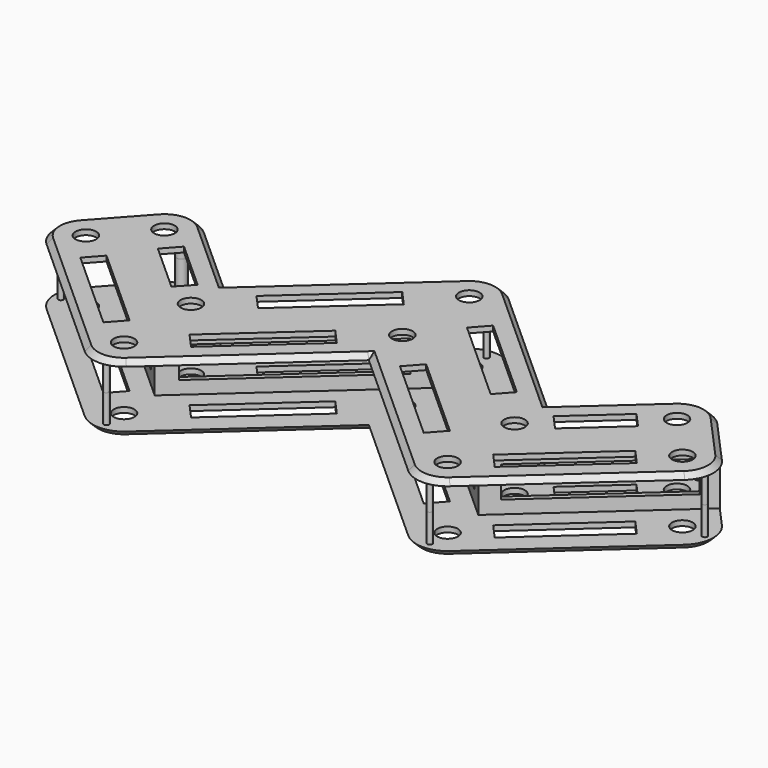
from build123d import *

# Parameters (mm, degrees)
F0_R           = 2
F0_R_2         = 1
F0_R_3         = 0.5
F1_DEPTH       = 6.5
F2_DEPTH       = 5.5
F3_W           = 30
F3_H           = 6
F4_DEPTH       = 1
F5_W           = 35
F5_H           = 6
F6_DEPTH       = 1.5
F7_W           = 35
F7_H           = 6
F8_DEPTH       = 1.5
F9_W           = 30
F9_H           = 6
F10_DEPTH      = 1.5
F11_R          = 6
F12_DEPTH      = 6.5
F13_T1_DEPTH   = 35.4024242658
F13_T3_DEPTH   = 35.4024242658
F13_T5_DEPTH   = 12
F13_T7_DEPTH   = 12
F13_T10_ANGLE  = 84
F13_T14_DEPTH  = 39.1692587222
F13_T19_DEPTH  = 39.1692587222
F13_T22_ANGLE  = 84
F13_T24_ANGLE  = 90
F13_T26_ANGLE  = 90
F13_T30_DEPTH  = 21.7668344564
F13_T35_DEPTH  = 39.1692587222
F13_T38_ANGLE  = 84
F13_T42_DEPTH  = 39.1692587222
F13_T47_DEPTH  = 21.7668344564
F13_T50_ANGLE  = 90
F13_T52_ANGLE  = 90
F13_T54_ANGLE  = 90
F13_T56_ANGLE  = 90
F13_T60_DEPTH  = 21.7668344564
F13_T65_DEPTH  = 39.1692587222
F13_T68_ANGLE  = 84
F13_T72_DEPTH  = 39.1692587222
F13_T77_DEPTH  = 21.7668344564
F13_T80_ANGLE  = 90
F13_T82_ANGLE  = 90
F13_T84_ANGLE  = 84
F13_T88_DEPTH  = 39.1692587222
F13_T93_DEPTH  = 39.1692587222
F13_T96_ANGLE  = 84
F13_T101_DEPTH = 39.1692587222
F13_T105_DEPTH = 39.1692587222
F13_T112_DEPTH = 21.7668344564
F13_T116_DEPTH = 39.1692587222
F13_T123_DEPTH = 39.1692587222
F13_T127_DEPTH = 21.7668344564
F13_T134_DEPTH = 21.7668344564
F13_T138_DEPTH = 39.1692587222
F13_T145_DEPTH = 39.1692587222
F13_T149_DEPTH = 21.7668344564
F13_T156_DEPTH = 39.1692587222
F13_T160_DEPTH = 39.1692587222


# Not quite as in the source:
# - a fillet or chamfer that OpenCascade refuses, or shapes differently, is made with other operations: its cross-section is extruded or revolved along the edge and cut away or added


with BuildPart() as f1:
    # F0 (on Top) → F1 (new body, symmetric)
    with BuildSketch(Plane.XY):
        Polygon((-49.9357291109, 33.0064397346), (-57.6307310841, 24.4602742417), (-31.2120826701, 0.6728163648), (0, 28.7763018319), (31.2120826701, 0.6728163648), (57.6307310841, 24.4602742417), (49.9357291109, 33.0064397346), (31.2120826701, 16.1475927553), (0, 44.2510782223), (-31.2120826701, 16.1475927553), align=None)
        with Locations((-31.2120826701, 8.0737963776)):
            Circle(F0_R, mode=Mode.SUBTRACT)
        with Locations((31.2120826701, 8.0737963776)):
            Circle(F0_R, mode=Mode.SUBTRACT)
        Polygon((-46.3710360561, 19.0317138545), (-43.6945136306, 22.0042931564), (-34.3115040691, 13.5557933995), (-37.0313460748, 10.6222192229), align=None, mode=Mode.SUBTRACT)
        with Locations((-49.8654209077, 29.0960744023)):
            Circle(F0_R_2, mode=Mode.SUBTRACT)
        with Locations((-49.4916437962, 24.5327871436)):
            Circle(F0_R, mode=Mode.SUBTRACT)
        Polygon((-22.4423732026, 13.2788127903), (-25.118895628, 16.2513920922), (-8.7697094675, 30.9722654321), (-6.0931870421, 27.9996861302), align=None, mode=Mode.SUBTRACT)
        Polygon((6.0931870421, 27.9996861302), (8.7697094675, 30.9722654321), (25.118895628, 16.2513920922), (22.4423732026, 13.2788127903), align=None, mode=Mode.SUBTRACT)
        Polygon((37.0092128356, 10.6022903648), (34.3326904102, 13.5748696667), (43.6361429708, 21.9517359782), (46.3126653962, 18.9791566763), align=None, mode=Mode.SUBTRACT)
        with Locations((49.4332731364, 24.4802299654)):
            Circle(F0_R, mode=Mode.SUBTRACT)
        with Locations((0, 36.1772818447)):
            Circle(F0_R, mode=Mode.SUBTRACT)
        with Locations((0, 40.3471924365)):
            Circle(F0_R_3, mode=Mode.SUBTRACT)
        with Locations((49.6616996825, 29.187746346)):
            Circle(F0_R_3, mode=Mode.SUBTRACT)
        Polygon((-31.2120826701, -0.6728163648), (-58.2998616904, 23.7171294162), (-65.9948636635, 15.1709639232), (-31.2120826701, -16.1475927553), (0, 11.9558927118), (31.2120826701, -16.1475927553), (65.9948636635, 15.1709639232), (58.2998616904, 23.7171294162), (31.2120826701, -0.6728163648), (0, 27.4306691023), align=None)
        with Locations((-31.124683097, -12.420842424)):
            Circle(F0_R_3, mode=Mode.SUBTRACT)
        with Locations((-31.2120826701, -8.0737963776)):
            Circle(F0_R, mode=Mode.SUBTRACT)
        Polygon((-53.6574585069, 9.4448453424), (-50.9809360815, 12.4174246443), (-35.0758352357, -1.9035924822), (-37.7523576611, -4.8761717841), align=None, mode=Mode.SUBTRACT)
        Polygon((-6.0931870421, 11.8520933749), (-22.4423732026, -2.868779965), (-25.118895628, 0.1037993369), (-8.7697094675, 14.8246726768), align=None, mode=Mode.SUBTRACT)
        with Locations((31.263994053, -12.4030448496)):
            Circle(F0_R_3, mode=Mode.SUBTRACT)
        with Locations((31.2120826701, -8.0737963776)):
            Circle(F0_R, mode=Mode.SUBTRACT)
        Polygon((22.4423732026, -2.868779965), (6.0931870421, 11.8520933749), (8.7697094675, 14.8246726768), (25.118895628, 0.1037993369), align=None, mode=Mode.SUBTRACT)
        Polygon((37.7523576611, -4.8761717841), (35.0758352357, -1.9035924822), (51.0113683193, 12.4448259544), (53.6878907447, 9.4722466525), align=None, mode=Mode.SUBTRACT)
        with Locations((-61.948928982, 15.132994391)):
            Circle(F0_R_3, mode=Mode.SUBTRACT)
        with Locations((-57.5212110725, 15.6150492379)):
            Circle(F0_R, mode=Mode.SUBTRACT)
        with Locations((0, 20.0296890894)):
            Circle(F0_R, mode=Mode.SUBTRACT)
        with Locations((57.5516433104, 15.6424505479)):
            Circle(F0_R, mode=Mode.SUBTRACT)
        with Locations((62.0999746025, 15.3564941138)):
            Circle(F0_R_3, mode=Mode.SUBTRACT)
        Polygon((-57.6307310841, 24.4602742417), (-57.9652963872, 24.0887018289), (-31.2120826701, 0), (0, 28.1034854671), (31.2120826701, 0), (57.9652963872, 24.0887018289), (57.6307310841, 24.4602742417), (31.2120826701, 0.6728163648), (0, 28.7763018319), (-31.2120826701, 0.6728163648), align=None)
        Polygon((-31.2120826701, 0), (-57.9652963872, 24.0887018289), (-58.2998616904, 23.7171294162), (-31.2120826701, -0.6728163648), (0, 27.4306691023), (31.2120826701, -0.6728163648), (58.2998616904, 23.7171294162), (57.9652963872, 24.0887018289), (31.2120826701, 0), (0, 28.1034854671), align=None)
    extrude(amount=F1_DEPTH, both=True)

    # F0 (on Top) → F2 (cut, symmetric)
    with BuildSketch(Plane.XY):
        Polygon((-49.9357291109, 33.0064397346), (-57.6307310841, 24.4602742417), (-31.2120826701, 0.6728163648), (0, 28.7763018319), (31.2120826701, 0.6728163648), (57.6307310841, 24.4602742417), (49.9357291109, 33.0064397346), (31.2120826701, 16.1475927553), (0, 44.2510782223), (-31.2120826701, 16.1475927553), align=None)
        with Locations((-31.2120826701, 8.0737963776)):
            Circle(F0_R, mode=Mode.SUBTRACT)
        with Locations((31.2120826701, 8.0737963776)):
            Circle(F0_R, mode=Mode.SUBTRACT)
        Polygon((-46.3710360561, 19.0317138545), (-43.6945136306, 22.0042931564), (-34.3115040691, 13.5557933995), (-37.0313460748, 10.6222192229), align=None, mode=Mode.SUBTRACT)
        with Locations((-49.8654209077, 29.0960744023)):
            Circle(F0_R_2, mode=Mode.SUBTRACT)
        with Locations((-49.4916437962, 24.5327871436)):
            Circle(F0_R, mode=Mode.SUBTRACT)
        Polygon((-22.4423732026, 13.2788127903), (-25.118895628, 16.2513920922), (-8.7697094675, 30.9722654321), (-6.0931870421, 27.9996861302), align=None, mode=Mode.SUBTRACT)
        Polygon((6.0931870421, 27.9996861302), (8.7697094675, 30.9722654321), (25.118895628, 16.2513920922), (22.4423732026, 13.2788127903), align=None, mode=Mode.SUBTRACT)
        Polygon((37.0092128356, 10.6022903648), (34.3326904102, 13.5748696667), (43.6361429708, 21.9517359782), (46.3126653962, 18.9791566763), align=None, mode=Mode.SUBTRACT)
        with Locations((49.4332731364, 24.4802299654)):
            Circle(F0_R, mode=Mode.SUBTRACT)
        with Locations((0, 36.1772818447)):
            Circle(F0_R, mode=Mode.SUBTRACT)
        with Locations((0, 40.3471924365)):
            Circle(F0_R_3, mode=Mode.SUBTRACT)
        with Locations((49.6616996825, 29.187746346)):
            Circle(F0_R_3, mode=Mode.SUBTRACT)
        Polygon((-31.2120826701, -0.6728163648), (-58.2998616904, 23.7171294162), (-65.9948636635, 15.1709639232), (-31.2120826701, -16.1475927553), (0, 11.9558927118), (31.2120826701, -16.1475927553), (65.9948636635, 15.1709639232), (58.2998616904, 23.7171294162), (31.2120826701, -0.6728163648), (0, 27.4306691023), align=None)
        with Locations((-31.124683097, -12.420842424)):
            Circle(F0_R_3, mode=Mode.SUBTRACT)
        with Locations((-31.2120826701, -8.0737963776)):
            Circle(F0_R, mode=Mode.SUBTRACT)
        Polygon((-53.6574585069, 9.4448453424), (-50.9809360815, 12.4174246443), (-35.0758352357, -1.9035924822), (-37.7523576611, -4.8761717841), align=None, mode=Mode.SUBTRACT)
        Polygon((-6.0931870421, 11.8520933749), (-22.4423732026, -2.868779965), (-25.118895628, 0.1037993369), (-8.7697094675, 14.8246726768), align=None, mode=Mode.SUBTRACT)
        with Locations((31.263994053, -12.4030448496)):
            Circle(F0_R_3, mode=Mode.SUBTRACT)
        with Locations((31.2120826701, -8.0737963776)):
            Circle(F0_R, mode=Mode.SUBTRACT)
        Polygon((22.4423732026, -2.868779965), (6.0931870421, 11.8520933749), (8.7697094675, 14.8246726768), (25.118895628, 0.1037993369), align=None, mode=Mode.SUBTRACT)
        Polygon((37.7523576611, -4.8761717841), (35.0758352357, -1.9035924822), (51.0113683193, 12.4448259544), (53.6878907447, 9.4722466525), align=None, mode=Mode.SUBTRACT)
        with Locations((-61.948928982, 15.132994391)):
            Circle(F0_R_3, mode=Mode.SUBTRACT)
        with Locations((-57.5212110725, 15.6150492379)):
            Circle(F0_R, mode=Mode.SUBTRACT)
        with Locations((0, 20.0296890894)):
            Circle(F0_R, mode=Mode.SUBTRACT)
        with Locations((57.5516433104, 15.6424505479)):
            Circle(F0_R, mode=Mode.SUBTRACT)
        with Locations((62.0999746025, 15.3564941138)):
            Circle(F0_R_3, mode=Mode.SUBTRACT)
    extrude(amount=F2_DEPTH, both=True, mode=Mode.SUBTRACT)

    # F3 (on face) → F4 (cut, symmetric)
    with BuildSketch(Plane(origin=(14.3093311198, -15.8921222204, 0), x_dir=(0.7431448255, 0.6691306064, 0), z_dir=(0.6691306064, -0.7431448255, 0))):
        with Locations((41.1773308546, 0)):
            Rectangle(F3_W, F3_H)
    extrude(amount=F4_DEPTH, both=True, mode=Mode.SUBTRACT)

    # F5 (on face) → F6 (cut, symmetric)
    with BuildSketch(Plane(origin=(14.3093311198, 15.8921222204, 0), x_dir=(-0.7431448255, 0.6691306064, 0), z_dir=(0.6691306064, 0.7431448255, 0))):
        with Locations((-2.5412207043, 0)):
            Rectangle(F5_W, F5_H)
    extrude(amount=F6_DEPTH, both=True, mode=Mode.SUBTRACT)

    # F7 (on face) → F8 (cut, symmetric)
    with BuildSketch(Plane(origin=(-13.6402005134, 15.148977395, 0), x_dir=(0.7431448255, 0.6691306064, 0), z_dir=(0.6691306064, -0.7431448255, 0))):
        with Locations((-2.5076098637, 0)):
            Rectangle(F7_W, F7_H)
    extrude(amount=F8_DEPTH, both=True, mode=Mode.SUBTRACT)

    # F9 (on face) → F10 (cut, symmetric)
    with BuildSketch(Plane(origin=(-14.3093311198, -15.8921222204, 0), x_dir=(0.7431448255, -0.6691306064, 0), z_dir=(-0.6691306064, -0.7431448255, 0))):
        with Locations((-40.9549903262, 0)):
            Rectangle(F9_W, F9_H)
    extrude(amount=F10_DEPTH, both=True, mode=Mode.SUBTRACT)

    # F11
    f11_edges = [f1.edges().sort_by_distance(p)[0] for p in [
        (49.935729, 33.00644, 6),
        (49.935729, 33.00644, -6),
        (0, 44.251078, -6),
        (0, 44.251078, 6),
        (-49.935729, 33.00644, -6),
        (-49.935729, 33.00644, 6),
        (-65.994864, 15.170964, -6),
        (-65.994864, 15.170964, 6),
        (-31.212083, -16.147593, 6),
        (-31.212083, -16.147593, -6),
        (31.212083, -16.147593, 6),
        (31.212083, -16.147593, -6),
        (65.994864, 15.170964, -6),
        (65.994864, 15.170964, 6),
    ]]
    fillet(f11_edges, radius=F11_R)

    # F0 (on Top) → F12 (join, symmetric)
    with BuildSketch(Plane.XY):
        with Locations((62.0999746025, 15.3564941138)):
            Circle(F0_R_3)
        with Locations((49.6616996825, 29.187746346)):
            Circle(F0_R_3)
        with Locations((0, 40.3471924365)):
            Circle(F0_R_3)
        with Locations((31.263994053, -12.4030448496)):
            Circle(F0_R_3)
        with Locations((-31.124683097, -12.420842424)):
            Circle(F0_R_3)
        with Locations((-49.8654209077, 29.0960744023)):
            Circle(F0_R_2)
        with Locations((-61.948928982, 15.132994391)):
            Circle(F0_R_3)
    extrude(amount=F12_DEPTH, both=True)

    # F13: chamfer of 1 on 34 edges, made by hand

    # F13_s2 → F13_t1 (cut)
    with BuildSketch(Plane(origin=(-39.5316616178, 35.5944679985, 0), x_dir=(0, 0, 1), z_dir=(0.7431448255, -0.6691306064, 0))):
        Polygon((6.5, 31.8849598027), (5.5, 32.8849598027), (6.5, 32.8849598027), align=None)
        Polygon((-6.5, 31.8849598027), (-5.5, 32.8849598027), (-6.5, 32.8849598027), align=None)
    extrude(amount=F13_T1_DEPTH, mode=Mode.SUBTRACT)

    # F13_s4 → F13_t3 (cut)
    with BuildSketch(Plane(origin=(13.2225332153, 11.9056223829, 0), x_dir=(0, 0, 1), z_dir=(0.7431448255, 0.6691306064, 0))):
        Polygon((6.5, 31.8849598027), (5.5, 32.8849598027), (6.5, 32.8849598027), align=None)
        Polygon((-6.5, 31.8849598027), (-5.5, 32.8849598027), (-6.5, 32.8849598027), align=None)
    extrude(amount=F13_T3_DEPTH, mode=Mode.SUBTRACT)

    # F13_s6 → F13_t5 (cut)
    with BuildSketch(Plane(origin=(17.9895494547, -19.9794187606, 0), x_dir=(0, 0, 1), z_dir=(-0.6691306064, 0.7431448255, 0))):
        Polygon((5.5, 59.1950977286), (6.5, 58.1950977286), (6.5, 59.1950977286), align=None)
        Polygon((-6.5, 58.1950977286), (-5.5, 59.1950977286), (-6.5, 59.1950977286), align=None)
    extrude(amount=F13_T5_DEPTH, mode=Mode.SUBTRACT)

    # F13_s8 → F13_t7 (cut)
    with BuildSketch(Plane(origin=(-9.9599821784, -11.0616808548, 0), x_dir=(0, 0, 1), z_dir=(-0.6691306064, -0.7431448255, 0))):
        Polygon((5.5, 59.1950977286), (6.5, 58.1950977286), (6.5, 59.1950977286), align=None)
        Polygon((-6.5, 58.1950977286), (-5.5, 59.1950977286), (-6.5, 59.1950977286), align=None)
    extrude(amount=F13_T7_DEPTH, mode=Mode.SUBTRACT)

    # F13_s9 → F13_t10 (revolve, cut)
    with BuildSketch(Plane(origin=(-13.2225332153, 11.9056223829, 0), x_dir=(0, 0, 1), z_dir=(-0.7431448255, 0.6691306064, 0))):
        Polygon((6.5, -31.8849598027), (5.5, -32.8849598027), (6.5, -32.8849598027), align=None)
    revolve(axis=Axis((-31.2120826701, -8.0737963776, 6.5), (0, 0, 1)), revolution_arc=F13_T10_ANGLE, mode=Mode.SUBTRACT)


with BuildPart() as f13_tool12:
    # F13_s13 → F13_t14 (new body)
    with BuildSketch(Plane(origin=(-21.2521004916, -19.1354772325, 0), x_dir=(0, 0, 1), z_dir=(0.7431448255, 0.6691306064, 0))):
        Polygon((6.5, -9.8849598027), (5.5, -8.8849598027), (6.5, -8.8849598027), align=None)
    extrude(amount=F13_T14_DEPTH)

    split(bisect_by=Plane(origin=(5.9451985403, 6.602811902, 0), x_dir=(0, 0, 1), z_dir=(-0.6691306064, -0.7431448255, 0)), keep=Keep.TOP)


with BuildPart() as f1_1:
    add(f1.part)

    # F13_t11: cut F13_tool12
    add(f13_tool12.part, mode=Mode.SUBTRACT)


with BuildPart() as f13_tool17:
    # F13_s18 → F13_t19 (new body)
    with BuildSketch(Plane(origin=(-7.8563314456, 7.0738726069, 0), x_dir=(0, 0, 1), z_dir=(0.7431448255, -0.6691306064, 0))):
        Polygon((6.5, -9.8849598027), (5.5, -8.8849598027), (6.5, -8.8849598027), align=None)
    extrude(amount=F13_T19_DEPTH)

    split(bisect_by=Plane(origin=(-5.9451985403, 6.602811902, 0), x_dir=(0, 0, 1), z_dir=(0.6691306064, -0.7431448255, 0)), keep=Keep.TOP)


with BuildPart() as f1_2:
    add(f1_1.part)

    # F13_t16: cut F13_tool17
    add(f13_tool17.part, mode=Mode.SUBTRACT)

    # F13_s21 → F13_t22 (revolve, cut)
    with BuildSketch(Plane(origin=(13.2225332153, 11.9056223829, 0), x_dir=(0, 0, 1), z_dir=(0.7431448255, 0.6691306064, 0))):
        Polygon((6.5, 31.8849598027), (5.5, 32.8849598027), (6.5, 32.8849598027), align=None)
    revolve(axis=Axis((31.2120826701, -8.0737963776, 6.5), (0, 0, -1)), revolution_arc=F13_T22_ANGLE, mode=Mode.SUBTRACT)

    # F13_s23 → F13_t24 (revolve, cut)
    with BuildSketch(Plane(origin=(17.9895494547, -19.9794187606, 0), x_dir=(0, 0, 1), z_dir=(-0.6691306064, 0.7431448255, 0))):
        Polygon((6.5, 58.1950977286), (5.5, 59.1950977286), (6.5, 59.1950977286), align=None)
    revolve(axis=Axis((57.5212110725, 15.6150492379, 6.5), (0, 0, -1)), revolution_arc=F13_T24_ANGLE, mode=Mode.SUBTRACT)

    # F13_s25 → F13_t26 (revolve, cut)
    with BuildSketch(Plane(origin=(9.9599821784, -11.0616808548, 0), x_dir=(0, 0, 1), z_dir=(0.6691306064, -0.7431448255, 0))):
        Polygon((6.5, -58.1950977286), (5.5, -59.1950977286), (6.5, -59.1950977286), align=None)
    revolve(axis=Axis((49.4916437962, 24.5327871436, 6.5), (0, 0, 1)), revolution_arc=F13_T26_ANGLE, mode=Mode.SUBTRACT)


with BuildPart() as f13_tool28:
    # F13_s29 → F13_t30 (new body)
    with BuildSketch(Plane(origin=(39.5316616178, 35.5944679985, 0), x_dir=(0, 0, 1), z_dir=(-0.7431448255, -0.6691306064, 0))):
        Polygon((6.5, -9.8849598027), (5.5, -8.8849598027), (6.5, -8.8849598027), align=None)
    extrude(amount=F13_T30_DEPTH)

    split(bisect_by=Plane(origin=(22.0043330929, 24.4382877134, 0), x_dir=(0, 0, 1), z_dir=(0.6691306064, 0.7431448255, 0)), keep=Keep.TOP)


with BuildPart() as f1_3:
    add(f1_2.part)

    # F13_t27: cut F13_tool28
    add(f13_tool28.part, mode=Mode.SUBTRACT)


with BuildPart() as f13_tool33:
    # F13_s34 → F13_t35 (new body)
    with BuildSketch(Plane(origin=(11.1188824824, -10.0114867553, 0), x_dir=(0, 0, 1), z_dir=(-0.7431448255, 0.6691306064, 0))):
        Polygon((6.5, 31.8849598027), (5.5, 32.8849598027), (6.5, 32.8849598027), align=None)
    extrude(amount=F13_T35_DEPTH)

    split(bisect_by=Plane(origin=(5.9451985403, -6.602811902, 0), x_dir=(0, 0, 1), z_dir=(-0.6691306064, 0.7431448255, 0)), keep=Keep.TOP)


with BuildPart() as f1_4:
    add(f1_3.part)

    # F13_t32: cut F13_tool33
    add(f13_tool33.part, mode=Mode.SUBTRACT)

    # F13_s37 → F13_t38 (revolve, cut)
    with BuildSketch(Plane(origin=(17.9895494547, 16.1978630841, 0), x_dir=(0, 0, 1), z_dir=(-0.7431448255, -0.6691306064, 0))):
        Polygon((6.5, 31.8849598027), (5.5, 32.8849598027), (6.5, 32.8849598027), align=None)
    revolve(axis=Axis((0, 36.1772818447, 6.5), (0, 0, -1)), revolution_arc=F13_T38_ANGLE, mode=Mode.SUBTRACT)


with BuildPart() as f13_tool40:
    # F13_s41 → F13_t42 (new body)
    with BuildSketch(Plane(origin=(17.9895494547, 16.1978630841, 0), x_dir=(0, 0, 1), z_dir=(-0.7431448255, -0.6691306064, 0))):
        Polygon((6.5, 31.8849598027), (5.5, 32.8849598027), (6.5, 32.8849598027), align=None)
    extrude(amount=F13_T42_DEPTH)

    split(bisect_by=Plane(origin=(-5.9451985403, -6.602811902, 0), x_dir=(0, 0, 1), z_dir=(0.6691306064, 0.7431448255, 0)), keep=Keep.TOP)


with BuildPart() as f1_5:
    add(f1_4.part)

    # F13_t39: cut F13_tool40
    add(f13_tool40.part, mode=Mode.SUBTRACT)


with BuildPart() as f13_tool45:
    # F13_s46 → F13_t47 (new body)
    with BuildSketch(Plane(origin=(-23.3557512245, 21.0296128602, 0), x_dir=(0, 0, 1), z_dir=(-0.7431448255, 0.6691306064, 0))):
        Polygon((6.5, -9.8849598027), (5.5, -8.8849598027), (6.5, -8.8849598027), align=None)
    extrude(amount=F13_T47_DEPTH)

    split(bisect_by=Plane(origin=(-22.0043330929, 24.4382877134, 0), x_dir=(0, 0, 1), z_dir=(-0.6691306064, 0.7431448255, 0)), keep=Keep.TOP)


with BuildPart() as f1_6:
    add(f1_5.part)

    # F13_t44: cut F13_tool45
    add(f13_tool45.part, mode=Mode.SUBTRACT)

    # F13_s49 → F13_t50 (revolve, cut)
    with BuildSketch(Plane(origin=(-9.9599821784, -11.0616808548, 0), x_dir=(0, 0, 1), z_dir=(-0.6691306064, -0.7431448255, 0))):
        Polygon((5.5, 59.1950977286), (6.5, 58.1950977286), (6.5, 59.1950977286), align=None)
    revolve(axis=Axis((-49.4916437962, 24.5327871436, 6.5), (0, 0, -1)), revolution_arc=F13_T50_ANGLE, mode=Mode.SUBTRACT)

    # F13_s51 → F13_t52 (revolve, cut)
    with BuildSketch(Plane(origin=(-17.9895494547, -19.9794187606, 0), x_dir=(0, 0, 1), z_dir=(0.6691306064, 0.7431448255, 0))):
        Polygon((6.5, -58.1950977286), (5.5, -59.1950977286), (6.5, -59.1950977286), align=None)
    revolve(axis=Axis((-57.5212110725, 15.6150492379, 6.5), (0, 0, 1)), revolution_arc=F13_T52_ANGLE, mode=Mode.SUBTRACT)

    # F13_s53 → F13_t54 (revolve, cut)
    with BuildSketch(Plane(origin=(17.9895494547, -19.9794187606, 0), x_dir=(0, 0, 1), z_dir=(-0.6691306064, 0.7431448255, 0))):
        Polygon((-6.5, 58.1950977286), (-5.5, 59.1950977286), (-6.5, 59.1950977286), align=None)
    revolve(axis=Axis((57.5212110725, 15.6150492379, -6.5), (0, 0, -1)), revolution_arc=F13_T54_ANGLE, mode=Mode.SUBTRACT)

    # F13_s55 → F13_t56 (revolve, cut)
    with BuildSketch(Plane(origin=(39.5316616178, 35.5944679985, 0), x_dir=(0, 0, 1), z_dir=(-0.7431448255, -0.6691306064, 0))):
        Polygon((-6.5, -9.8849598027), (-5.5, -8.8849598027), (-6.5, -8.8849598027), align=None)
    revolve(axis=Axis((49.4916437962, 24.5327871436, -6.5), (0, 0, -1)), revolution_arc=F13_T56_ANGLE, mode=Mode.SUBTRACT)


with BuildPart() as f13_tool58:
    # F13_s59 → F13_t60 (new body)
    with BuildSketch(Plane(origin=(39.5316616178, 35.5944679985, 0), x_dir=(0, 0, 1), z_dir=(-0.7431448255, -0.6691306064, 0))):
        Polygon((-6.5, -9.8849598027), (-5.5, -8.8849598027), (-6.5, -8.8849598027), align=None)
    extrude(amount=F13_T60_DEPTH)

    split(bisect_by=Plane(origin=(22.0043330929, 24.4382877134, 0), x_dir=(0, 0, 1), z_dir=(0.6691306064, 0.7431448255, 0)), keep=Keep.TOP)


with BuildPart() as f1_7:
    add(f1_6.part)

    # F13_t57: cut F13_tool58
    add(f13_tool58.part, mode=Mode.SUBTRACT)


with BuildPart() as f13_tool63:
    # F13_s64 → F13_t65 (new body)
    with BuildSketch(Plane(origin=(11.1188824824, -10.0114867553, 0), x_dir=(0, 0, 1), z_dir=(-0.7431448255, 0.6691306064, 0))):
        Polygon((-6.5, 31.8849598027), (-5.5, 32.8849598027), (-6.5, 32.8849598027), align=None)
    extrude(amount=F13_T65_DEPTH)

    split(bisect_by=Plane(origin=(5.9451985403, -6.602811902, 0), x_dir=(0, 0, 1), z_dir=(-0.6691306064, 0.7431448255, 0)), keep=Keep.TOP)


with BuildPart() as f1_8:
    add(f1_7.part)

    # F13_t62: cut F13_tool63
    add(f13_tool63.part, mode=Mode.SUBTRACT)

    # F13_s67 → F13_t68 (revolve, cut)
    with BuildSketch(Plane(origin=(17.9895494547, 16.1978630841, 0), x_dir=(0, 0, 1), z_dir=(-0.7431448255, -0.6691306064, 0))):
        Polygon((-5.5, 32.8849598027), (-6.5, 31.8849598027), (-6.5, 32.8849598027), align=None)
    revolve(axis=Axis((0, 36.1772818447, -6.5), (0, 0, -1)), revolution_arc=F13_T68_ANGLE, mode=Mode.SUBTRACT)


with BuildPart() as f13_tool70:
    # F13_s71 → F13_t72 (new body)
    with BuildSketch(Plane(origin=(17.9895494547, 16.1978630841, 0), x_dir=(0, 0, 1), z_dir=(-0.7431448255, -0.6691306064, 0))):
        Polygon((-5.5, 32.8849598027), (-6.5, 31.8849598027), (-6.5, 32.8849598027), align=None)
    extrude(amount=F13_T72_DEPTH)

    split(bisect_by=Plane(origin=(-5.9451985403, -6.602811902, 0), x_dir=(0, 0, 1), z_dir=(0.6691306064, 0.7431448255, 0)), keep=Keep.TOP)


with BuildPart() as f1_9:
    add(f1_8.part)

    # F13_t69: cut F13_tool70
    add(f13_tool70.part, mode=Mode.SUBTRACT)


with BuildPart() as f13_tool75:
    # F13_s76 → F13_t77 (new body)
    with BuildSketch(Plane(origin=(-23.3557512245, 21.0296128602, 0), x_dir=(0, 0, 1), z_dir=(-0.7431448255, 0.6691306064, 0))):
        Polygon((-5.5, -8.8849598027), (-6.5, -9.8849598027), (-6.5, -8.8849598027), align=None)
    extrude(amount=F13_T77_DEPTH)

    split(bisect_by=Plane(origin=(-22.0043330929, 24.4382877134, 0), x_dir=(0, 0, 1), z_dir=(-0.6691306064, 0.7431448255, 0)), keep=Keep.TOP)


with BuildPart() as f1_10:
    add(f1_9.part)

    # F13_t74: cut F13_tool75
    add(f13_tool75.part, mode=Mode.SUBTRACT)

    # F13_s79 → F13_t80 (revolve, cut)
    with BuildSketch(Plane(origin=(-39.5316616178, 35.5944679985, 0), x_dir=(0, 0, 1), z_dir=(0.7431448255, -0.6691306064, 0))):
        Polygon((-6.5, 9.8849598027), (-5.5, 8.8849598027), (-6.5, 8.8849598027), align=None)
    revolve(axis=Axis((-49.4916437962, 24.5327871436, -6.5), (0, 0, 1)), revolution_arc=F13_T80_ANGLE, mode=Mode.SUBTRACT)

    # F13_s81 → F13_t82 (revolve, cut)
    with BuildSketch(Plane(origin=(-17.9895494547, -19.9794187606, 0), x_dir=(0, 0, 1), z_dir=(0.6691306064, 0.7431448255, 0))):
        Polygon((-6.5, -58.1950977286), (-5.5, -59.1950977286), (-6.5, -59.1950977286), align=None)
    revolve(axis=Axis((-57.5212110725, 15.6150492379, -6.5), (0, 0, 1)), revolution_arc=F13_T82_ANGLE, mode=Mode.SUBTRACT)

    # F13_s83 → F13_t84 (revolve, cut)
    with BuildSketch(Plane(origin=(-13.2225332153, 11.9056223829, 0), x_dir=(0, 0, 1), z_dir=(-0.7431448255, 0.6691306064, 0))):
        Polygon((-6.5, -31.8849598027), (-5.5, -32.8849598027), (-6.5, -32.8849598027), align=None)
    revolve(axis=Axis((-31.2120826701, -8.0737963776, -6.5), (0, 0, 1)), revolution_arc=F13_T84_ANGLE, mode=Mode.SUBTRACT)


with BuildPart() as f13_tool86:
    # F13_s87 → F13_t88 (new body)
    with BuildSketch(Plane(origin=(-21.2521004916, -19.1354772325, 0), x_dir=(0, 0, 1), z_dir=(0.7431448255, 0.6691306064, 0))):
        Polygon((-6.5, -9.8849598027), (-5.5, -8.8849598027), (-6.5, -8.8849598027), align=None)
    extrude(amount=F13_T88_DEPTH)

    split(bisect_by=Plane(origin=(5.9451985403, 6.602811902, 0), x_dir=(0, 0, 1), z_dir=(-0.6691306064, -0.7431448255, 0)), keep=Keep.TOP)


with BuildPart() as f1_11:
    add(f1_10.part)

    # F13_t85: cut F13_tool86
    add(f13_tool86.part, mode=Mode.SUBTRACT)


with BuildPart() as f13_tool91:
    # F13_s92 → F13_t93 (new body)
    with BuildSketch(Plane(origin=(-7.8563314456, 7.0738726069, 0), x_dir=(0, 0, 1), z_dir=(0.7431448255, -0.6691306064, 0))):
        Polygon((-6.5, -9.8849598027), (-5.5, -8.8849598027), (-6.5, -8.8849598027), align=None)
    extrude(amount=F13_T93_DEPTH)

    split(bisect_by=Plane(origin=(-5.9451985403, 6.602811902, 0), x_dir=(0, 0, 1), z_dir=(0.6691306064, -0.7431448255, 0)), keep=Keep.TOP)


with BuildPart() as f1_12:
    add(f1_11.part)

    # F13_t90: cut F13_tool91
    add(f13_tool91.part, mode=Mode.SUBTRACT)

    # F13_s95 → F13_t96 (revolve, cut)
    with BuildSketch(Plane(origin=(21.2521004916, -19.1354772325, 0), x_dir=(0, 0, 1), z_dir=(-0.7431448255, 0.6691306064, 0))):
        Polygon((-6.5, 9.8849598027), (-5.5, 8.8849598027), (-6.5, 8.8849598027), align=None)
    revolve(axis=Axis((31.2120826701, -8.0737963776, -6.5), (0, 0, 1)), revolution_arc=F13_T96_ANGLE, mode=Mode.SUBTRACT)


with BuildPart() as f13_tool99:
    # F13_s100 → F13_t101 (new body)
    with BuildSketch(Plane(origin=(-21.2521004916, -19.1354772325, 0), x_dir=(0, 0, 1), z_dir=(0.7431448255, 0.6691306064, 0))):
        Polygon((6.5, -9.8849598027), (5.5, -8.8849598027), (6.5, -8.8849598027), align=None)
    extrude(amount=F13_T101_DEPTH)

    split(bisect_by=Plane(origin=(5.9451985403, 6.602811902, 0), x_dir=(0, 0, 1), z_dir=(0.6691306064, 0.7431448255, 0)), keep=Keep.TOP)


with BuildPart() as f13_tool103:
    # F13_s104 → F13_t105 (new body)
    with BuildSketch(Plane(origin=(-7.8563314456, 7.0738726069, 0), x_dir=(0, 0, 1), z_dir=(0.7431448255, -0.6691306064, 0))):
        Polygon((6.5, -9.8849598027), (5.5, -8.8849598027), (6.5, -8.8849598027), align=None)
    extrude(amount=F13_T105_DEPTH)

    split(bisect_by=Plane(origin=(-5.9451985403, 6.602811902, 0), x_dir=(0, 0, 1), z_dir=(-0.6691306064, 0.7431448255, 0)), keep=Keep.TOP)


with BuildPart() as f13_tool99_1:
    add(f13_tool99.part)

    # F13_t107: intersect F13_tool103
    add(f13_tool103.part, mode=Mode.INTERSECT)


with BuildPart() as f1_13:
    add(f1_12.part)

    # F13_t97: cut F13_tool99
    add(f13_tool99_1.part, mode=Mode.SUBTRACT)


with BuildPart() as f13_tool110:
    # F13_s111 → F13_t112 (new body)
    with BuildSketch(Plane(origin=(39.5316616178, 35.5944679985, 0), x_dir=(0, 0, 1), z_dir=(-0.7431448255, -0.6691306064, 0))):
        Polygon((6.5, -9.8849598027), (5.5, -8.8849598027), (6.5, -8.8849598027), align=None)
    extrude(amount=F13_T112_DEPTH)

    split(bisect_by=Plane(origin=(22.0043330929, 24.4382877134, 0), x_dir=(0, 0, 1), z_dir=(-0.6691306064, -0.7431448255, 0)), keep=Keep.TOP)


with BuildPart() as f13_tool114:
    # F13_s115 → F13_t116 (new body)
    with BuildSketch(Plane(origin=(11.1188824824, -10.0114867553, 0), x_dir=(0, 0, 1), z_dir=(-0.7431448255, 0.6691306064, 0))):
        Polygon((6.5, 31.8849598027), (5.5, 32.8849598027), (6.5, 32.8849598027), align=None)
    extrude(amount=F13_T116_DEPTH)

    split(bisect_by=Plane(origin=(5.9451985403, -6.602811902, 0), x_dir=(0, 0, 1), z_dir=(0.6691306064, -0.7431448255, 0)), keep=Keep.TOP)


with BuildPart() as f13_tool110_1:
    add(f13_tool110.part)

    # F13_t118: intersect F13_tool114
    add(f13_tool114.part, mode=Mode.INTERSECT)


with BuildPart() as f1_14:
    add(f1_13.part)

    # F13_t108: cut F13_tool110
    add(f13_tool110_1.part, mode=Mode.SUBTRACT)


with BuildPart() as f13_tool121:
    # F13_s122 → F13_t123 (new body)
    with BuildSketch(Plane(origin=(17.9895494547, 16.1978630841, 0), x_dir=(0, 0, 1), z_dir=(-0.7431448255, -0.6691306064, 0))):
        Polygon((6.5, 31.8849598027), (5.5, 32.8849598027), (6.5, 32.8849598027), align=None)
    extrude(amount=F13_T123_DEPTH)

    split(bisect_by=Plane(origin=(-5.9451985403, -6.602811902, 0), x_dir=(0, 0, 1), z_dir=(-0.6691306064, -0.7431448255, 0)), keep=Keep.TOP)


with BuildPart() as f13_tool125:
    # F13_s126 → F13_t127 (new body)
    with BuildSketch(Plane(origin=(-23.3557512245, 21.0296128602, 0), x_dir=(0, 0, 1), z_dir=(-0.7431448255, 0.6691306064, 0))):
        Polygon((6.5, -9.8849598027), (5.5, -8.8849598027), (6.5, -8.8849598027), align=None)
    extrude(amount=F13_T127_DEPTH)

    split(bisect_by=Plane(origin=(-22.0043330929, 24.4382877134, 0), x_dir=(0, 0, 1), z_dir=(0.6691306064, -0.7431448255, 0)), keep=Keep.TOP)


with BuildPart() as f13_tool121_1:
    add(f13_tool121.part)

    # F13_t129: intersect F13_tool125
    add(f13_tool125.part, mode=Mode.INTERSECT)


with BuildPart() as f1_15:
    add(f1_14.part)

    # F13_t119: cut F13_tool121
    add(f13_tool121_1.part, mode=Mode.SUBTRACT)


with BuildPart() as f13_tool132:
    # F13_s133 → F13_t134 (new body)
    with BuildSketch(Plane(origin=(39.5316616178, 35.5944679985, 0), x_dir=(0, 0, 1), z_dir=(-0.7431448255, -0.6691306064, 0))):
        Polygon((-6.5, -9.8849598027), (-5.5, -8.8849598027), (-6.5, -8.8849598027), align=None)
    extrude(amount=F13_T134_DEPTH)

    split(bisect_by=Plane(origin=(22.0043330929, 24.4382877134, 0), x_dir=(0, 0, 1), z_dir=(-0.6691306064, -0.7431448255, 0)), keep=Keep.TOP)


with BuildPart() as f13_tool136:
    # F13_s137 → F13_t138 (new body)
    with BuildSketch(Plane(origin=(11.1188824824, -10.0114867553, 0), x_dir=(0, 0, 1), z_dir=(-0.7431448255, 0.6691306064, 0))):
        Polygon((-6.5, 31.8849598027), (-5.5, 32.8849598027), (-6.5, 32.8849598027), align=None)
    extrude(amount=F13_T138_DEPTH)

    split(bisect_by=Plane(origin=(5.9451985403, -6.602811902, 0), x_dir=(0, 0, 1), z_dir=(0.6691306064, -0.7431448255, 0)), keep=Keep.TOP)


with BuildPart() as f13_tool132_1:
    add(f13_tool132.part)

    # F13_t140: intersect F13_tool136
    add(f13_tool136.part, mode=Mode.INTERSECT)


with BuildPart() as f1_16:
    add(f1_15.part)

    # F13_t130: cut F13_tool132
    add(f13_tool132_1.part, mode=Mode.SUBTRACT)


with BuildPart() as f13_tool143:
    # F13_s144 → F13_t145 (new body)
    with BuildSketch(Plane(origin=(17.9895494547, 16.1978630841, 0), x_dir=(0, 0, 1), z_dir=(-0.7431448255, -0.6691306064, 0))):
        Polygon((-5.5, 32.8849598027), (-6.5, 31.8849598027), (-6.5, 32.8849598027), align=None)
    extrude(amount=F13_T145_DEPTH)

    split(bisect_by=Plane(origin=(-5.9451985403, -6.602811902, 0), x_dir=(0, 0, 1), z_dir=(-0.6691306064, -0.7431448255, 0)), keep=Keep.TOP)


with BuildPart() as f13_tool147:
    # F13_s148 → F13_t149 (new body)
    with BuildSketch(Plane(origin=(-23.3557512245, 21.0296128602, 0), x_dir=(0, 0, 1), z_dir=(-0.7431448255, 0.6691306064, 0))):
        Polygon((-5.5, -8.8849598027), (-6.5, -9.8849598027), (-6.5, -8.8849598027), align=None)
    extrude(amount=F13_T149_DEPTH)

    split(bisect_by=Plane(origin=(-22.0043330929, 24.4382877134, 0), x_dir=(0, 0, 1), z_dir=(0.6691306064, -0.7431448255, 0)), keep=Keep.TOP)


with BuildPart() as f13_tool143_1:
    add(f13_tool143.part)

    # F13_t151: intersect F13_tool147
    add(f13_tool147.part, mode=Mode.INTERSECT)


with BuildPart() as f1_17:
    add(f1_16.part)

    # F13_t141: cut F13_tool143
    add(f13_tool143_1.part, mode=Mode.SUBTRACT)


with BuildPart() as f13_tool154:
    # F13_s155 → F13_t156 (new body)
    with BuildSketch(Plane(origin=(-21.2521004916, -19.1354772325, 0), x_dir=(0, 0, 1), z_dir=(0.7431448255, 0.6691306064, 0))):
        Polygon((-6.5, -9.8849598027), (-5.5, -8.8849598027), (-6.5, -8.8849598027), align=None)
    extrude(amount=F13_T156_DEPTH)

    split(bisect_by=Plane(origin=(5.9451985403, 6.602811902, 0), x_dir=(0, 0, 1), z_dir=(0.6691306064, 0.7431448255, 0)), keep=Keep.TOP)


with BuildPart() as f13_tool158:
    # F13_s159 → F13_t160 (new body)
    with BuildSketch(Plane(origin=(-7.8563314456, 7.0738726069, 0), x_dir=(0, 0, 1), z_dir=(0.7431448255, -0.6691306064, 0))):
        Polygon((-6.5, -9.8849598027), (-5.5, -8.8849598027), (-6.5, -8.8849598027), align=None)
    extrude(amount=F13_T160_DEPTH)

    split(bisect_by=Plane(origin=(-5.9451985403, 6.602811902, 0), x_dir=(0, 0, 1), z_dir=(-0.6691306064, 0.7431448255, 0)), keep=Keep.TOP)


with BuildPart() as f13_tool154_1:
    add(f13_tool154.part)

    # F13_t162: intersect F13_tool158
    add(f13_tool158.part, mode=Mode.INTERSECT)


with BuildPart() as f1_18:
    add(f1_17.part)

    # F13_t152: cut F13_tool154
    add(f13_tool154_1.part, mode=Mode.SUBTRACT)


solid = f1_18.part
